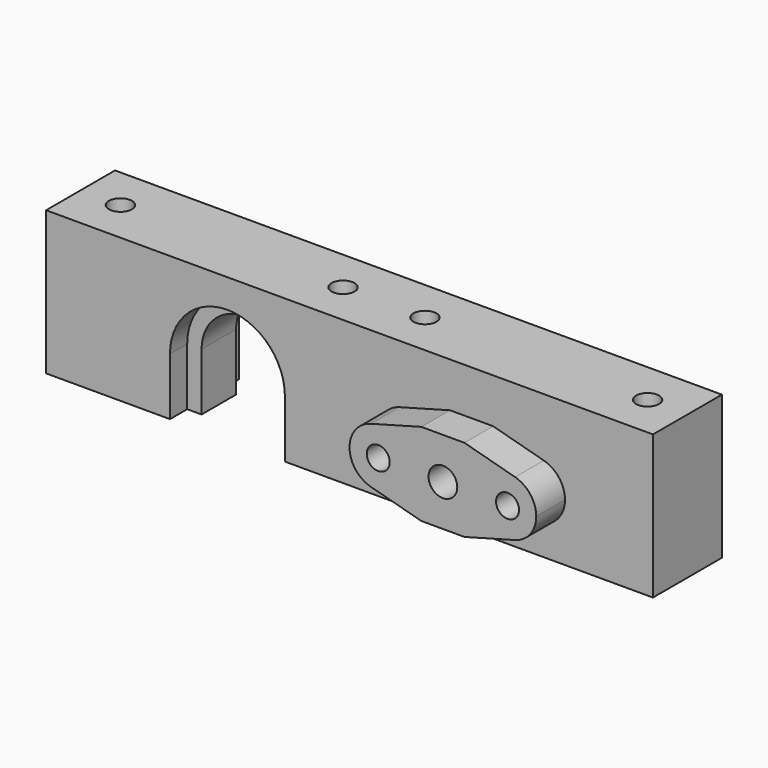
from build123d import *

# Parameters (mm, degrees)
F0_W      = 84.5
F0_H      = 12
F1_DEPTH  = 20
F3_DEPTH  = 3
F4_DEPTH  = 25
F5_R      = 1.6
F5_W      = 6
F5_H      = 11.54
F5_R_2    = 2
F6_DEPTH  = 5
F7_DEPTH  = 25
F8_R      = 2
F8_R_2    = 1.6
F9_DEPTH  = 10
F10_R     = 1.6
F11_DEPTH = 25
F12_R     = 1.6
F13_DEPTH = 12
F14_DEPTH = 10


# Not quite as in the source:
# - a pattern or mirror of a feature is missing from the dataset's text; its kind, count and spacing are read off the source's solid


with BuildPart() as f1:
    # F0 (on Top) → F1 (new body)
    with BuildSketch(Plane.XY):
        Rectangle(F0_W, F0_H)
    extrude(amount=F1_DEPTH)

    # F2 (on face) → F3 (cut)
    with BuildSketch(Plane(origin=(0, 6, 0), x_dir=(-1, 0, 0), z_dir=(0, 1, 0))):
        with BuildLine():
            ThreePointArc((11, 8), (17, 2), (23, 8))
            ThreePointArc((23, 8), (17, 14), (11, 8))
        make_face()
        with BuildLine():
            Line((23, 2.7084973779), (23, 8))
            ThreePointArc((23, 8), (17, 2), (11, 8))
            Line((11, 8), (11, 2.7084973779))
            ThreePointArc((11, 2.7084973779), (13.7084973779, 0.7084973779), (17, 0))
            ThreePointArc((17, 0), (20.2915026221, 0.7084973779), (23, 2.7084973779))
        make_face()
        with BuildLine():
            Line((23, 0), (23, 2.7084973779))
            ThreePointArc((23, 2.7084973779), (20.2915026221, 0.7084973779), (17, 0))
            Line((17, 0), (23, 0))
        make_face()
        with BuildLine():
            ThreePointArc((25, 8), (24.4833147735, 5.1715728753), (23, 2.7084973779))
            Line((23, 2.7084973779), (23, 0))
            Line((23, 0), (25, 0))
            Line((25, 0), (25, 8))
        make_face()
        with BuildLine():
            ThreePointArc((17, 0), (13.7084973779, 0.7084973779), (11, 2.7084973779))
            Line((11, 2.7084973779), (11, 0))
            Line((11, 0), (17, 0))
        make_face()
        with BuildLine():
            Line((11, 0), (11, 2.7084973779))
            ThreePointArc((11, 2.7084973779), (9.5166852265, 5.1715728753), (9, 8))
            Line((9, 8), (9, 0))
            Line((9, 0), (11, 0))
        make_face()
        with BuildLine():
            ThreePointArc((11, 8), (17, 14), (23, 8))
            Line((23, 8), (23, 2.7084973779))
            ThreePointArc((23, 2.7084973779), (24.4833147735, 5.1715728753), (25, 8))
            ThreePointArc((25, 8), (17, 16), (9, 8))
            ThreePointArc((9, 8), (9.5166852265, 5.1715728753), (11, 2.7084973779))
            Line((11, 2.7084973779), (11, 8))
        make_face()
    f3 = extrude(amount=-F3_DEPTH, mode=Mode.SUBTRACT)

    # F3_copies: F3 across plane
    add(f3.mirror(Plane(origin=(0, 0, 0), x_dir=(0, 0, -1), z_dir=(0, -1, 0))), mode=Mode.SUBTRACT)

    # F2 (on face) → F4 (cut)
    with BuildSketch(Plane(origin=(0, 6, 0), x_dir=(-1, 0, 0), z_dir=(0, 1, 0))):
        with BuildLine():
            Line((23, 2.7084973779), (23, 8))
            ThreePointArc((23, 8), (17, 2), (11, 8))
            Line((11, 8), (11, 2.7084973779))
            ThreePointArc((11, 2.7084973779), (13.7084973779, 0.7084973779), (17, 0))
            ThreePointArc((17, 0), (20.2915026221, 0.7084973779), (23, 2.7084973779))
        make_face()
        with BuildLine():
            Line((23, 0), (23, 2.7084973779))
            ThreePointArc((23, 2.7084973779), (20.2915026221, 0.7084973779), (17, 0))
            Line((17, 0), (23, 0))
        make_face()
        with BuildLine():
            ThreePointArc((17, 0), (13.7084973779, 0.7084973779), (11, 2.7084973779))
            Line((11, 2.7084973779), (11, 0))
            Line((11, 0), (17, 0))
        make_face()
        with BuildLine():
            ThreePointArc((11, 8), (17, 2), (23, 8))
            ThreePointArc((23, 8), (17, 14), (11, 8))
        make_face()
    extrude(amount=-F4_DEPTH, mode=Mode.SUBTRACT)

    # F5 (on face) → F6 (join)
    with BuildSketch(Plane.XZ.offset(6)):
        with BuildLine():
            ThreePointArc((12, 8), (10.430589025, 11.1768281338), (6.9538815041, 11.8607817981))
            ThreePointArc((6.9538815041, 11.8607817981), (4, 8), (6.9538815041, 4.1392182019))
            ThreePointArc((6.9538815041, 4.1392182019), (10.430589025, 4.8231718662), (12, 8))
        make_face()
        with Locations((8, 8)):
            Circle(F5_R, mode=Mode.SUBTRACT)
        with BuildLine():
            Line((14, 2.23), (14, 13.77))
            Line((14, 13.77), (6.9538815041, 11.8607817981))
            ThreePointArc((6.9538815041, 11.8607817981), (10.430589025, 11.1768281338), (12, 8))
            ThreePointArc((12, 8), (10.430589025, 4.8231718662), (6.9538815041, 4.1392182019))
            Line((6.9538815041, 4.1392182019), (14, 2.23))
        make_face()
        with Locations((17, 8)):
            Rectangle(F5_W, F5_H)
        with Locations((17, 8)):
            Circle(F5_R_2, mode=Mode.SUBTRACT)
        with BuildLine():
            Line((27.0461184959, 11.8607817981), (20, 13.77))
            Line((20, 13.77), (20, 2.23))
            Line((20, 2.23), (27.0461184959, 4.1392182019))
            ThreePointArc((27.0461184959, 4.1392182019), (22, 8), (27.0461184959, 11.8607817981))
        make_face()
        with BuildLine():
            ThreePointArc((30, 8), (29.1768281338, 10.430589025), (27.0461184959, 11.8607817981))
            ThreePointArc((27.0461184959, 11.8607817981), (22, 8), (27.0461184959, 4.1392182019))
            ThreePointArc((27.0461184959, 4.1392182019), (29.1768281338, 5.569410975), (30, 8))
        make_face()
        with Locations((26, 8)):
            Circle(F5_R, mode=Mode.SUBTRACT)
    extrude(amount=F6_DEPTH)

    # F5 (on face) → F7 (cut)
    with BuildSketch(Plane.XZ.offset(6)):
        with Locations((8, 8)):
            Circle(F5_R)
        with Locations((17, 8)):
            Circle(F5_R_2)
        with Locations((26, 8)):
            Circle(F5_R)
    extrude(amount=-F7_DEPTH, mode=Mode.SUBTRACT)

    # F8 (on face) → F9 (cut)
    with BuildSketch(Plane(origin=(0, 6, 0), x_dir=(-1, 0, 0), z_dir=(0, 1, 0))):
        with BuildLine():
            Line((-6.9538815041, 11.8607817981), (-14, 13.77))
            Line((-14, 13.77), (-20, 13.77))
            Line((-20, 13.77), (-27.0461184959, 11.8607817981))
            ThreePointArc((-27.0461184959, 11.8607817981), (-23.569410975, 11.1768281338), (-22, 8))
            ThreePointArc((-22, 8), (-23.569410975, 4.8231718662), (-27.0461184959, 4.1392182019))
            Line((-27.0461184959, 4.1392182019), (-20, 2.23))
            Line((-20, 2.23), (-14, 2.23))
            Line((-14, 2.23), (-6.9538815041, 4.1392182019))
            ThreePointArc((-6.9538815041, 4.1392182019), (-12, 8), (-6.9538815041, 11.8607817981))
        make_face()
        with Locations((-17, 8)):
            Circle(F8_R, mode=Mode.SUBTRACT)
        with BuildLine():
            ThreePointArc((-4, 8), (-4.8231718662, 10.430589025), (-6.9538815041, 11.8607817981))
            ThreePointArc((-6.9538815041, 11.8607817981), (-12, 8), (-6.9538815041, 4.1392182019))
            ThreePointArc((-6.9538815041, 4.1392182019), (-4.8231718662, 5.569410975), (-4, 8))
        make_face()
        with Locations((-8, 8)):
            Circle(F8_R_2, mode=Mode.SUBTRACT)
        with BuildLine():
            ThreePointArc((-22, 8), (-23.569410975, 11.1768281338), (-27.0461184959, 11.8607817981))
            ThreePointArc((-27.0461184959, 11.8607817981), (-29.1768281338, 10.430589025), (-30, 8))
            ThreePointArc((-30, 8), (-29.1768281338, 5.569410975), (-27.0461184959, 4.1392182019))
            ThreePointArc((-27.0461184959, 4.1392182019), (-23.569410975, 4.8231718662), (-22, 8))
        make_face()
        with Locations((-26, 8)):
            Circle(F8_R_2, mode=Mode.SUBTRACT)
    extrude(amount=-F9_DEPTH, mode=Mode.SUBTRACT)

    # F10 (on face) → F11 (cut)
    with BuildSketch(Plane.XY.offset(20)):
        with Locations((-36.7, 0)):
            Circle(F10_R)
        with Locations((-5.7, 0)):
            Circle(F10_R)
        with Locations((5.7, 0)):
            Circle(F10_R)
        with Locations((36.7, 0)):
            Circle(F10_R)
    extrude(amount=-F11_DEPTH, mode=Mode.SUBTRACT)

    # F12 (on face) → F13 (cut)
    with BuildSketch(Plane(origin=(0, 6, 0), x_dir=(-1, 0, 0), z_dir=(0, 1, 0))):
        Polygon((-6.5680812925, 10.4061605963), (-9.3678368482, 10.443158275), (-10.7997555557, 8.0369976787), (-9.4319187075, 5.5938394037), (-6.6321631518, 5.556841725), (-5.2002444443, 7.9630023213), align=None)
        with Locations((-8, 8)):
            Circle(F12_R, mode=Mode.SUBTRACT)
        Polygon((-28.7997555557, 7.9630023213), (-27.3678368482, 5.556841725), (-24.5680812925, 5.5938394037), (-23.2002444443, 8.0369976787), (-24.6321631518, 10.443158275), (-27.4319187075, 10.4061605963), align=None)
        with Locations((-26, 8)):
            Circle(F12_R, mode=Mode.SUBTRACT)
    extrude(amount=-F13_DEPTH, mode=Mode.SUBTRACT)

    # F8 (on face) → F14 (cut)
    with BuildSketch(Plane(origin=(0, 6, 0), x_dir=(-1, 0, 0), z_dir=(0, 1, 0))):
        with BuildLine():
            ThreePointArc((-8.3944853395, 0), (-7.0789353021, 1.8624403356), (-6.9538815041, 4.1392182019))
            Line((-6.9538815041, 4.1392182019), (-14, 2.23))
            Line((-14, 2.23), (-20, 2.23))
            Line((-20, 2.23), (-27.0461184959, 4.1392182019))
            ThreePointArc((-27.0461184959, 4.1392182019), (-29.1768281338, 5.569410975), (-30, 8))
            Line((-30, 8), (-30, 0))
            Line((-30, 0), (-8.3944853395, 0))
        make_face()
    extrude(amount=-F14_DEPTH, mode=Mode.SUBTRACT)


solid = f1.part
